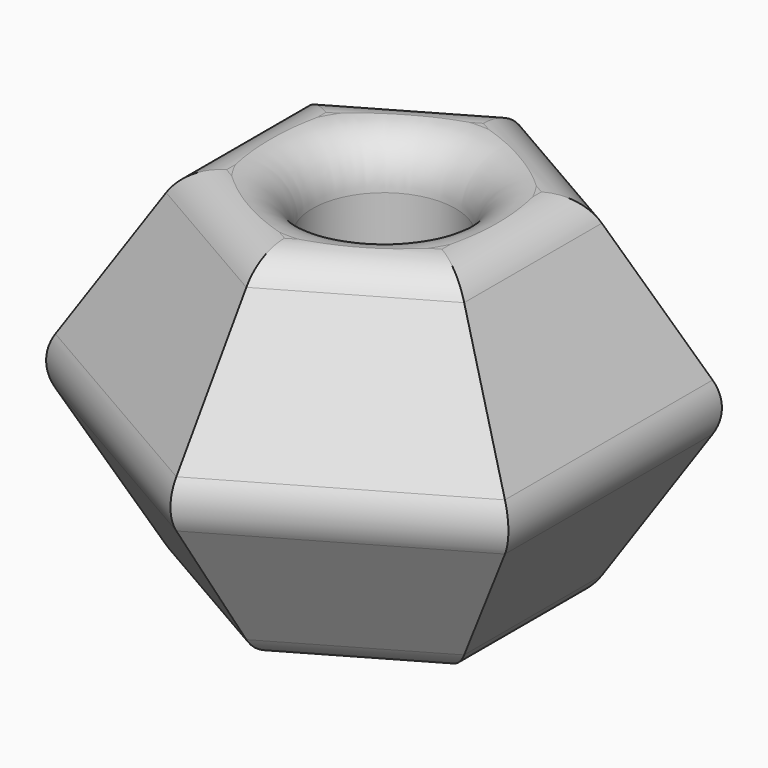
from build123d import *

# Parameters (mm, degrees)
F1_DEPTH     = 7.5
F1_TAPER     = 30
F2_R         = 3
F3_DEPTH     = 15.0010001
F4_T1_DEPTH  = 17.3205080757
F4_T3_DEPTH  = 12.3205080757
F4_T5_DEPTH  = 17.3205080757
F4_T7_DEPTH  = 12.3205080757
F4_T9_DEPTH  = 12.3205080757
F4_T11_DEPTH = 12.3205080757
F4_T13_DEPTH = 12.3205080757
F4_T15_DEPTH = 17.3205080757
F4_T17_DEPTH = 17.3205080757
F4_T19_DEPTH = 17.3205080757


# Not quite as in the source:
# - a fillet or chamfer that OpenCascade refuses, or shapes differently, is made with other operations: its cross-section is extruded or revolved along the edge and cut away or added


with BuildPart() as f1:
    # F0 (on Top) → F1 (new body, symmetric)
    with BuildSketch(Plane.XY):
        Polygon((10, -5.7735026919), (10, 5.7735026919), (0, 11.5470053838), (-10, 5.7735026919), (-10, -5.7735026919), (0, -11.5470053838), align=None)
    extrude(amount=F1_DEPTH, both=True, taper=F1_TAPER)

    # F2 (on face) → F3 (cut, through all)
    with BuildSketch(Plane.XY.offset(7.5)):
        Circle(F2_R)
    extrude(amount=-F3_DEPTH, mode=Mode.SUBTRACT)

    # F4: fillet of radius 2 on 21 edges, made by hand

    # F4_s2 → F4_t1 (cut)
    with BuildSketch(Plane.XZ.offset(-8.6602540378)):
        with BuildLine():
            ThreePointArc((9.4226497308, -1), (9.6905989232, 0), (9.4226497308, 1))
            Line((9.4226497308, 1), (10, 0))
            Line((10, 0), (9.4226497308, -1))
        make_face()
        with BuildLine():
            ThreePointArc((-9.4226497308, -1), (-9.6905989232, 0), (-9.4226497308, 1))
            Line((-9.4226497308, 1), (-10, 0))
            Line((-10, 0), (-9.4226497308, -1))
        make_face()
    extrude(amount=F4_T1_DEPTH, mode=Mode.SUBTRACT)

    # F4_s4 → F4_t3 (cut)
    with BuildSketch(Plane.XZ.offset(-6.1602540378)):
        with BuildLine():
            ThreePointArc((6.2472232503, -6.5), (5.5151724427, -7.2320508076), (4.5151724427, -7.5))
            Line((4.5151724427, -7.5), (5.6698729811, -7.5))
            Line((5.6698729811, -7.5), (6.2472232503, -6.5))
        make_face()
        with BuildLine():
            ThreePointArc((6.2472232503, 6.5), (5.5151724427, 7.2320508076), (4.5151724427, 7.5))
            Line((4.5151724427, 7.5), (5.6698729811, 7.5))
            Line((5.6698729811, 7.5), (6.2472232503, 6.5))
        make_face()
        with BuildLine():
            ThreePointArc((-4.5151724427, -7.5), (-5.5151724427, -7.2320508076), (-6.2472232503, -6.5))
            Line((-6.2472232503, -6.5), (-5.6698729811, -7.5))
            Line((-5.6698729811, -7.5), (-4.5151724427, -7.5))
        make_face()
        with BuildLine():
            ThreePointArc((-4.5151724427, 7.5), (-5.5151724427, 7.2320508076), (-6.2472232503, 6.5))
            Line((-6.2472232503, 6.5), (-5.6698729811, 7.5))
            Line((-5.6698729811, 7.5), (-4.5151724427, 7.5))
        make_face()
    extrude(amount=F4_T3_DEPTH, mode=Mode.SUBTRACT)

    # F4_s6 → F4_t5 (cut)
    with BuildSketch(Plane(origin=(7.5, -4.3301270189, 0), x_dir=(0, 0, 1), z_dir=(-0.8660254038, 0.5, 0))):
        with BuildLine():
            ThreePointArc((-1, 9.4226497308), (0, 9.6905989232), (1, 9.4226497308))
            Line((1, 9.4226497308), (0, 10))
            Line((0, 10), (-1, 9.4226497308))
        make_face()
    extrude(amount=F4_T5_DEPTH, mode=Mode.SUBTRACT)

    # F4_s8 → F4_t7 (cut)
    with BuildSketch(Plane(origin=(5.3349364905, -3.0801270189, 0), x_dir=(0, 0, 1), z_dir=(-0.8660254038, 0.5, 0))):
        with BuildLine():
            ThreePointArc((-6.5, 6.2472232503), (-7.2320508076, 5.5151724427), (-7.5, 4.5151724427))
            Line((-7.5, 4.5151724427), (-7.5, 5.6698729811))
            Line((-7.5, 5.6698729811), (-6.5, 6.2472232503))
        make_face()
        with BuildLine():
            ThreePointArc((6.5, 6.2472232503), (7.2320508076, 5.5151724427), (7.5, 4.5151724427))
            Line((7.5, 4.5151724427), (7.5, 5.6698729811))
            Line((7.5, 5.6698729811), (6.5, 6.2472232503))
        make_face()
    extrude(amount=F4_T7_DEPTH, mode=Mode.SUBTRACT)

    # F4_s10 → F4_t9 (cut)
    with BuildSketch(Plane(origin=(-5.3349364905, -3.0801270189, 0), x_dir=(0, 0, 1), z_dir=(0.8660254038, 0.5, 0))):
        with BuildLine():
            ThreePointArc((-7.5, 4.5151724427), (-7.2320508076, 5.5151724427), (-6.5, 6.2472232503))
            Line((-6.5, 6.2472232503), (-7.5, 5.6698729811))
            Line((-7.5, 5.6698729811), (-7.5, 4.5151724427))
        make_face()
        with BuildLine():
            ThreePointArc((6.5, 6.2472232503), (7.2320508076, 5.5151724427), (7.5, 4.5151724427))
            Line((7.5, 4.5151724427), (7.5, 5.6698729811))
            Line((7.5, 5.6698729811), (6.5, 6.2472232503))
        make_face()
    extrude(amount=F4_T9_DEPTH, mode=Mode.SUBTRACT)

    # F4_s12 → F4_t11 (cut)
    with BuildSketch(Plane(origin=(-5.3349364905, 3.0801270189, 0), x_dir=(0, 0, 1), z_dir=(0.8660254038, -0.5, 0))):
        with BuildLine():
            ThreePointArc((-7.5, 4.5151724427), (-7.2320508076, 5.5151724427), (-6.5, 6.2472232503))
            Line((-6.5, 6.2472232503), (-7.5, 5.6698729811))
            Line((-7.5, 5.6698729811), (-7.5, 4.5151724427))
        make_face()
        with BuildLine():
            ThreePointArc((7.5, 4.5151724427), (7.2320508076, 5.5151724427), (6.5, 6.2472232503))
            Line((6.5, 6.2472232503), (7.5, 5.6698729811))
            Line((7.5, 5.6698729811), (7.5, 4.5151724427))
        make_face()
    extrude(amount=F4_T11_DEPTH, mode=Mode.SUBTRACT)

    # F4_s14 → F4_t13 (cut)
    with BuildSketch(Plane(origin=(5.3349364905, 3.0801270189, 0), x_dir=(0, 0, 1), z_dir=(-0.8660254038, -0.5, 0))):
        with BuildLine():
            ThreePointArc((-7.5, 4.5151724427), (-7.2320508076, 5.5151724427), (-6.5, 6.2472232503))
            Line((-6.5, 6.2472232503), (-7.5, 5.6698729811))
            Line((-7.5, 5.6698729811), (-7.5, 4.5151724427))
        make_face()
        with BuildLine():
            ThreePointArc((7.5, 4.5151724427), (7.2320508076, 5.5151724427), (6.5, 6.2472232503))
            Line((6.5, 6.2472232503), (7.5, 5.6698729811))
            Line((7.5, 5.6698729811), (7.5, 4.5151724427))
        make_face()
    extrude(amount=F4_T13_DEPTH, mode=Mode.SUBTRACT)

    # F4_s16 → F4_t15 (cut)
    with BuildSketch(Plane(origin=(-7.5, -4.3301270189, 0), x_dir=(0, 0, 1), z_dir=(0.8660254038, 0.5, 0))):
        with BuildLine():
            ThreePointArc((-1, 9.4226497308), (0, 9.6905989232), (1, 9.4226497308))
            Line((1, 9.4226497308), (0, 10))
            Line((0, 10), (-1, 9.4226497308))
        make_face()
    extrude(amount=F4_T15_DEPTH, mode=Mode.SUBTRACT)

    # F4_s18 → F4_t17 (cut)
    with BuildSketch(Plane(origin=(7.5, 4.3301270189, 0), x_dir=(0, 0, 1), z_dir=(-0.8660254038, -0.5, 0))):
        with BuildLine():
            ThreePointArc((-1, 9.4226497308), (0, 9.6905989232), (1, 9.4226497308))
            Line((1, 9.4226497308), (0, 10))
            Line((0, 10), (-1, 9.4226497308))
        make_face()
    extrude(amount=F4_T17_DEPTH, mode=Mode.SUBTRACT)

    # F4_s20 → F4_t19 (cut)
    with BuildSketch(Plane(origin=(-7.5, 4.3301270189, 0), x_dir=(0, 0, 1), z_dir=(0.8660254038, -0.5, 0))):
        with BuildLine():
            ThreePointArc((-1, 9.4226497308), (0, 9.6905989232), (1, 9.4226497308))
            Line((1, 9.4226497308), (0, 10))
            Line((0, 10), (-1, 9.4226497308))
        make_face()
    extrude(amount=F4_T19_DEPTH, mode=Mode.SUBTRACT)

    # F4_s21 → F4_t22 (revolve, cut)
    with BuildSketch(Plane.XZ):
        with BuildLine():
            ThreePointArc((5, -7.5), (3.5857864376, -6.9142135624), (3, -5.5))
            Line((3, -5.5), (3, -7.5))
            Line((3, -7.5), (5, -7.5))
        make_face()
    revolve(axis=Axis((0, 0, -7.5), (0, 0, 1)), mode=Mode.SUBTRACT)

    # F4_s23 → F4_t24 (revolve, cut)
    with BuildSketch(Plane.XZ):
        with BuildLine():
            ThreePointArc((5, 7.5), (3.5857864376, 6.9142135624), (3, 5.5))
            Line((3, 5.5), (3, 7.5))
            Line((3, 7.5), (5, 7.5))
        make_face()
    revolve(axis=Axis((0, 0, 7.5), (0, 0, 1)), mode=Mode.SUBTRACT)


solid = f1.part
